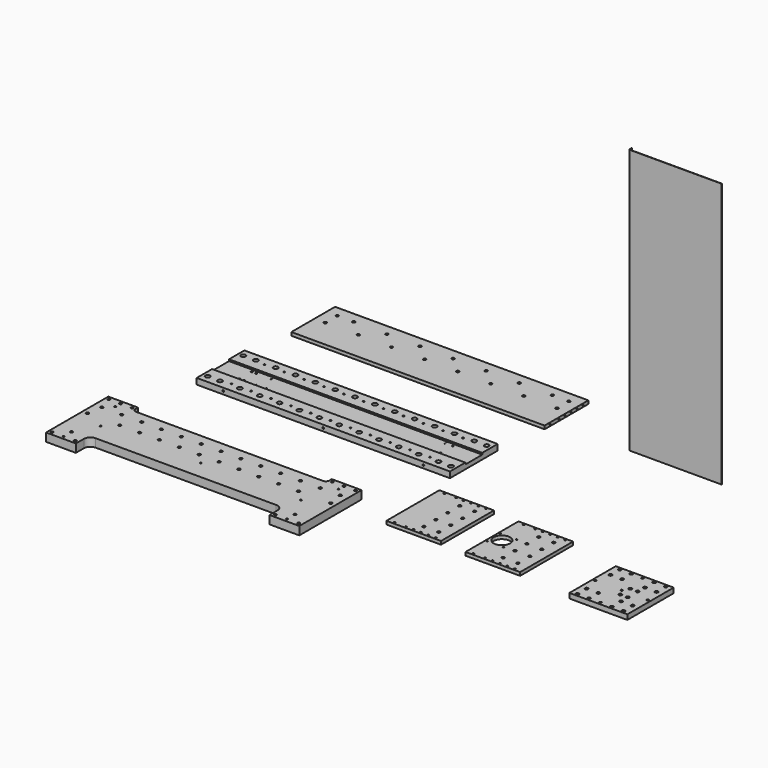
from build123d import *

# Parameters (mm, degrees)
F0_W            = 765
F0_H            = 180
F0_R            = 2.5
F1_DEPTH        = 18
F0_H_2          = 165
F2_DEPTH        = 10
F4_R            = 2.1
F5_DEPTH        = 15
F6_R            = 2.1
F7_DEPTH        = 15
F0_W_2          = 165
F0_H_3          = 200
F0_R_2          = 2.65
F8_DEPTH        = 10
F9_DEPTH        = 10
F0_W_3          = 175
F0_H_4          = 175
F0_R_3          = 4.75
F0_R_4          = 3.35
F0_R_5          = 3
F10_DEPTH       = 15
F11_DEPTH       = 9
F12_W           = 765
F12_H           = 64
F12_R           = 2.5
F13_DEPTH       = 5
F14_DEPTH       = 9.3
F15_DEPTH       = 25
F17_D           = 7.5
F18_D           = 5
F19_DEPTH       = 800
F20_D           = 50
F21_D           = 4.2
F22_D           = 8.4
F23_D           = 8.4
F25_D           = 8.4
F25_CBORE_D     = 14
F25_CBORE_DEPTH = 9
F27_D           = 8.4
F27_CBORE_D     = 14
F27_CBORE_DEPTH = 11
F28_D           = 8.4
F30_D           = 2.5
F32_D           = 5
F32_DEPTH       = 12
F32_TIP         = 1.5021515476
F33_D           = 4.99
F33_DEPTH       = 10
F33_TIP         = 1.4991472445


# Not quite as in the source:
# - a feature names something its author has since deleted; it is built from what else it names


with BuildPart() as f1:
    # F0 (on Top) → F1 (new body)
    with BuildSketch(Plane.XY):
        with Locations((62.1241629124, -27)):
            Rectangle(F0_W, F0_H)
        with Locations((-237.8758370876, -89.5)):
            Circle(F0_R, mode=Mode.SUBTRACT)
        with Locations((-244.3758370876, -50)):
            Circle(F0_R, mode=Mode.SUBTRACT)
        with Locations((-231.3758370876, -50)):
            Circle(F0_R, mode=Mode.SUBTRACT)
        with Locations((-244.3758370876, -4)):
            Circle(F0_R, mode=Mode.SUBTRACT)
        with Locations((-231.3758370876, -4)):
            Circle(F0_R, mode=Mode.SUBTRACT)
        with Locations((-177.8758370876, -89.5)):
            Circle(F0_R, mode=Mode.SUBTRACT)
        with Locations((-117.8758370876, -89.5)):
            Circle(F0_R, mode=Mode.SUBTRACT)
        with Locations((-57.8758370876, -89.5)):
            Circle(F0_R, mode=Mode.SUBTRACT)
        with Locations((-237.8758370876, 35.5)):
            Circle(F0_R, mode=Mode.SUBTRACT)
        with Locations((-177.8758370876, 35.5)):
            Circle(F0_R, mode=Mode.SUBTRACT)
        with Locations((-117.8758370876, 35.5)):
            Circle(F0_R, mode=Mode.SUBTRACT)
        with Locations((-57.8758370876, 35.5)):
            Circle(F0_R, mode=Mode.SUBTRACT)
        with Locations((2.1241629124, -89.5)):
            Circle(F0_R, mode=Mode.SUBTRACT)
        with Locations((62.1241629124, -89.5)):
            Circle(F0_R, mode=Mode.SUBTRACT)
        with Locations((122.1241629124, -89.5)):
            Circle(F0_R, mode=Mode.SUBTRACT)
        with Locations((182.1241629124, -89.5)):
            Circle(F0_R, mode=Mode.SUBTRACT)
        with Locations((242.1241629124, -89.5)):
            Circle(F0_R, mode=Mode.SUBTRACT)
        with Locations((302.1241629124, -89.5)):
            Circle(F0_R, mode=Mode.SUBTRACT)
        with Locations((362.1241629124, -89.5)):
            Circle(F0_R, mode=Mode.SUBTRACT)
        with Locations((362.6241629124, -50)):
            Circle(F0_R, mode=Mode.SUBTRACT)
        with Locations((362.6241629124, -4)):
            Circle(F0_R, mode=Mode.SUBTRACT)
        with Locations((2.1241629124, 35.5)):
            Circle(F0_R, mode=Mode.SUBTRACT)
        with Locations((62.1241629124, 35.5)):
            Circle(F0_R, mode=Mode.SUBTRACT)
        with Locations((122.1241629124, 35.5)):
            Circle(F0_R, mode=Mode.SUBTRACT)
        with Locations((182.1241629124, 35.5)):
            Circle(F0_R, mode=Mode.SUBTRACT)
        with Locations((242.1241629124, 35.5)):
            Circle(F0_R, mode=Mode.SUBTRACT)
        with Locations((302.1241629124, 35.5)):
            Circle(F0_R, mode=Mode.SUBTRACT)
        with Locations((362.1241629124, 35.5)):
            Circle(F0_R, mode=Mode.SUBTRACT)
    extrude(amount=F1_DEPTH)

    # F12 (on face) → F13 (cut)
    with BuildSketch(Plane.XY.offset(18)):
        with Locations((62.1241629124, -27)):
            Rectangle(F12_W, F12_H)
        with Locations((-244.3758370876, -50)):
            Circle(F12_R, mode=Mode.SUBTRACT)
        with Locations((-231.3758370876, -50)):
            Circle(F12_R, mode=Mode.SUBTRACT)
        with Locations((362.6241629124, -50)):
            Circle(F12_R, mode=Mode.SUBTRACT)
        with Locations((-244.3758370876, -4)):
            Circle(F12_R, mode=Mode.SUBTRACT)
        with Locations((-231.3758370876, -4)):
            Circle(F12_R, mode=Mode.SUBTRACT)
        with Locations((362.6241629124, -4)):
            Circle(F12_R, mode=Mode.SUBTRACT)
    extrude(amount=-F13_DEPTH, mode=Mode.SUBTRACT)

    # F25 (through all)
    with Locations(Plane.XY.offset(18)):
        with Locations((-305.3758370876, 40.5), (-305.3758370876, -94.5), (-267.8758370876, 40.5), (-267.8758370876, -94.5), (-207.8758370876, 40.5), (-207.8758370876, -94.5), (-147.8758370876, 40.5), (-147.8758370876, -94.5), (-87.8758370876, 40.5), (-87.8758370876, -94.5), (-27.8758370876, 40.5), (-27.8758370876, -94.5), (32.1241629124, -94.5), (92.1241629124, -94.5), (152.1241629124, -94.5), (212.1241629124, -94.5), (32.1241629124, 40.5), (92.1241629124, 40.5), (152.1241629124, 40.5), (212.1241629124, 40.5), (272.1241629124, 40.5), (332.1241629124, 40.5), (392.1241629124, 40.5), (429.6241629124, 40.5), (272.1241629124, -94.5), (332.1241629124, -94.5), (392.1241629124, -94.5), (429.6241629124, -94.5)):
            CounterBoreHole(F25_D / 2, F25_CBORE_D / 2, F25_CBORE_DEPTH)

    # F30 (through all)
    with Locations(Plane.XY.offset(13)):
        with Locations((-185.3758370876, 1), (-185.3758370876, -6), (-195.3758370876, -48), (-195.3758370876, -55), (-165.3758370876, -47.9999991988), (-165.3758370876, -55), (339.6241629124, 1), (339.6241629124, -6)):
            Hole(F30_D / 2)

    # F32
    with Locations(Plane.XZ.offset(117)):
        with Locations((-240.3758370876, 9), (62.1241629124, 9), (364.6241629124, 9)):
            Hole(F32_D / 2, depth=F32_DEPTH)
            with Locations((0, 0, -(F32_DEPTH + F32_TIP / 2))):  # 118° drill point
                Cone(0, F32_D / 2, F32_TIP, mode=Mode.SUBTRACT)


with BuildPart() as f2:
    # F0 (on Top) → F2 (new body)
    with BuildSketch(Plane.XY):
        with Locations((80.4346650839, 300.0778406858)):
            Rectangle(F0_W, F0_H_2)
    extrude(amount=F2_DEPTH)

    # F4 (on face) → F5 (cut)
    with BuildSketch(Plane.YZ.offset(462.9346650839)):
        with Locations((237.5778406858, 5)):
            Circle(F4_R)
        with Locations((272.5778406858, 5)):
            Circle(F4_R)
        with Locations((295.0778406858, 5)):
            Circle(F4_R)
        with Locations((317.5778406858, 5)):
            Circle(F4_R)
        with Locations((340.0778406858, 5)):
            Circle(F4_R)
        with Locations((362.5778406858, 5)):
            Circle(F4_R)
    extrude(amount=-F5_DEPTH, mode=Mode.SUBTRACT)

    # F6 (on face) → F7 (cut)
    with BuildSketch(Plane(origin=(-302.0653349161, 0, 0), x_dir=(0, -1, 0), z_dir=(-1, 0, 0))):
        with Locations((-237.5778406858, 5)):
            Circle(F6_R)
        with Locations((-272.5778406858, 5)):
            Circle(F6_R)
        with Locations((-295.0778406858, 5)):
            Circle(F6_R)
        with Locations((-317.5778406858, 5)):
            Circle(F6_R)
        with Locations((-340.0778406858, 5)):
            Circle(F6_R)
        with Locations((-362.5778406858, 5)):
            Circle(F6_R)
    extrude(amount=-F7_DEPTH, mode=Mode.SUBTRACT)

    # F28 (through all)
    with Locations(Plane.XY.offset(10)):
        with Locations((-269.5653349161, 350.0778406858), (-269.5653349161, 305.0778406858), (-219.5653349161, 350.0778406858), (-169.5653349161, 305.0778406858), (-119.5653349161, 350.0778406858), (-69.5653349161, 305.0778406858), (-19.5653349161, 350.0778406858), (30.4346650839, 305.0778406858), (80.4346650839, 350.0778406858), (130.4346650839, 305.0778406858), (180.4346650839, 350.0778406858), (230.4346650839, 305.0778406858), (280.4346650839, 350.0778406858), (330.4346650839, 305.0778406858), (380.4346650839, 350.0778406858), (430.4346650839, 350.0778406858), (430.4346650839, 305.0778406858)):
            Hole(F28_D / 2)


with BuildPart() as f8:
    # F0 (on Top) → F8 (new body)
    with BuildSketch(Plane.XY):
        with Locations((557.9147299131, -295.5082142353)):
            Rectangle(F0_W_2, F0_H_3)
        with Locations((495.4147299131, -390.5082142353)):
            Circle(F0_R_2, mode=Mode.SUBTRACT)
        with Locations((530.4147299131, -390.5082142353)):
            Circle(F0_R_2, mode=Mode.SUBTRACT)
        with Locations((552.9147299131, -390.5082142353)):
            Circle(F0_R_2, mode=Mode.SUBTRACT)
        with Locations((575.4147299131, -390.5082142353)):
            Circle(F0_R_2, mode=Mode.SUBTRACT)
        with Locations((597.9147299131, -390.5082142353)):
            Circle(F0_R_2, mode=Mode.SUBTRACT)
        with Locations((620.4147299131, -390.5082142353)):
            Circle(F0_R_2, mode=Mode.SUBTRACT)
        with Locations((495.4147299131, -200.5082142353)):
            Circle(F0_R_2, mode=Mode.SUBTRACT)
        with Locations((530.4147299131, -200.5082142353)):
            Circle(F0_R_2, mode=Mode.SUBTRACT)
        with Locations((552.9147299131, -200.5082142353)):
            Circle(F0_R_2, mode=Mode.SUBTRACT)
        with Locations((575.4147299131, -200.5082142353)):
            Circle(F0_R_2, mode=Mode.SUBTRACT)
        with Locations((597.9147299131, -200.5082142353)):
            Circle(F0_R_2, mode=Mode.SUBTRACT)
        with Locations((620.4147299131, -200.5082142353)):
            Circle(F0_R_2, mode=Mode.SUBTRACT)
    extrude(amount=F8_DEPTH)

    # F23 (through all)
    with Locations(Plane(origin=(0, 0, 0), x_dir=(1, 0, 0), z_dir=(0, 0, -1))):
        with Locations((607.9147299131, 228.0082142353), (562.9147299131, 228.0082142353), (607.9147299131, 273.0082142353), (562.9147299131, 273.0082142353), (607.9147299131, 318.0082142353), (562.9147299131, 318.0082142353), (607.9147299131, 363.0082142353), (562.9147299131, 363.0082142353)):
            Hole(F23_D / 2)


with BuildPart() as f9:
    # F0 (on Top) → F9 (new body)
    with BuildSketch(Plane.XY):
        Polygon((720.5080483251, -303.1488111544), (720.5080483251, -403.1488111544), (885.5080483251, -403.1488111544), (885.5080483251, -203.1488111544), (720.5080483251, -203.1488111544), align=None)
        with Locations((740.5080483251, -398.1488111544)):
            Circle(F0_R_2, mode=Mode.SUBTRACT)
        with Locations((775.5080483251, -398.1488111544)):
            Circle(F0_R_2, mode=Mode.SUBTRACT)
        with Locations((798.0080483251, -398.1488111544)):
            Circle(F0_R_2, mode=Mode.SUBTRACT)
        with Locations((820.5080483251, -398.1488111544)):
            Circle(F0_R_2, mode=Mode.SUBTRACT)
        with Locations((843.0080483251, -398.1488111544)):
            Circle(F0_R_2, mode=Mode.SUBTRACT)
        with Locations((865.5080483251, -398.1488111544)):
            Circle(F0_R_2, mode=Mode.SUBTRACT)
        with Locations((740.5080483251, -208.1488111544)):
            Circle(F0_R_2, mode=Mode.SUBTRACT)
        with Locations((775.5080483251, -208.1488111544)):
            Circle(F0_R_2, mode=Mode.SUBTRACT)
        with Locations((798.0080483251, -208.1488111544)):
            Circle(F0_R_2, mode=Mode.SUBTRACT)
        with Locations((820.5080483251, -208.1488111544)):
            Circle(F0_R_2, mode=Mode.SUBTRACT)
        with Locations((843.0080483251, -208.1488111544)):
            Circle(F0_R_2, mode=Mode.SUBTRACT)
        with Locations((865.5080483251, -208.1488111544)):
            Circle(F0_R_2, mode=Mode.SUBTRACT)
    extrude(amount=F9_DEPTH)

    # F20 (through all)
    with Locations(Plane(origin=(0, 0, 0), x_dir=(1, 0, 0), z_dir=(0, 0, -1))):
        with Locations((750.5080483251, 303.1488111544)):
            Hole(F20_D / 2)

    # F21 (through all)
    with Locations(Plane(origin=(0, 0, 0), x_dir=(1, 0, 0), z_dir=(0, 0, -1))):
        with Locations((775.2567856666, 278.4000738129), (725.7593109836, 278.4000738129), (775.2567856666, 327.8975484959), (725.7593109836, 327.8975484959)):
            Hole(F21_D / 2)

    # F22 (through all)
    with Locations(Plane(origin=(0, 0, 0), x_dir=(1, 0, 0), z_dir=(0, 0, -1))):
        with Locations((853.0080483251, 235.6488111544), (808.0080483251, 235.6488111544), (808.0080483251, 280.6488111544), (853.0080483251, 280.6488111544), (853.0080483251, 325.6488111544), (808.0080483251, 325.6488111544), (808.0080483251, 370.6488111544), (853.0080483251, 370.6488111544)):
            Hole(F22_D / 2)


with BuildPart() as f10:
    # F0 (on Top) → F10 (new body)
    with BuildSketch(Plane.XY):
        with Locations((1136.3020181656, -333.5187590122)):
            Rectangle(F0_W_3, F0_H_4)
        with Locations((1066.8020181656, -413.5187590122)):
            Circle(F0_R_3, mode=Mode.SUBTRACT)
        with Locations((1101.8020181656, -413.5187590122)):
            Circle(F0_R_3, mode=Mode.SUBTRACT)
        with Locations((1136.3020181656, -413.0187590122)):
            Circle(F0_R_4, mode=Mode.SUBTRACT)
        with Locations((1170.8020181656, -413.5187590122)):
            Circle(F0_R_3, mode=Mode.SUBTRACT)
        with Locations((1205.8020181656, -413.5187590122)):
            Circle(F0_R_3, mode=Mode.SUBTRACT)
        with Locations((1066.8020181656, -378.5187590122)):
            Circle(F0_R_3, mode=Mode.SUBTRACT)
        with Locations((1101.8020181656, -378.5187590122)):
            Circle(F0_R_3, mode=Mode.SUBTRACT)
        with Locations((1056.8020181656, -333.5187590122)):
            Circle(F0_R_4, mode=Mode.SUBTRACT)
        with Locations((1170.8020181656, -378.5187590122)):
            Circle(F0_R_3, mode=Mode.SUBTRACT)
        with Locations((1205.8020181656, -378.5187590122)):
            Circle(F0_R_3, mode=Mode.SUBTRACT)
        with Locations((1147.8020181656, -352.5187590122)):
            Circle(F0_R_3, mode=Mode.SUBTRACT)
        with Locations((1169.8020181656, -352.5187590122)):
            Circle(F0_R_3, mode=Mode.SUBTRACT)
        with Locations((1136.3020181656, -333.5187590122)):
            Circle(F0_R_5, mode=Mode.SUBTRACT)
        with Locations((1215.8020181656, -333.5187590122)):
            Circle(F0_R_4, mode=Mode.SUBTRACT)
        with Locations((1066.8020181656, -288.5187590122)):
            Circle(F0_R_3, mode=Mode.SUBTRACT)
        with Locations((1101.8020181656, -288.5187590122)):
            Circle(F0_R_3, mode=Mode.SUBTRACT)
        with Locations((1147.8020181656, -314.5187590122)):
            Circle(F0_R_3, mode=Mode.SUBTRACT)
        with Locations((1169.8020181656, -314.5187590122)):
            Circle(F0_R_3, mode=Mode.SUBTRACT)
        with Locations((1170.8020181656, -288.5187590122)):
            Circle(F0_R_3, mode=Mode.SUBTRACT)
        with Locations((1205.8020181656, -288.5187590122)):
            Circle(F0_R_3, mode=Mode.SUBTRACT)
        with Locations((1066.8020181656, -253.5187590122)):
            Circle(F0_R_3, mode=Mode.SUBTRACT)
        with Locations((1101.8020181656, -253.5187590122)):
            Circle(F0_R_3, mode=Mode.SUBTRACT)
        with Locations((1136.3020181656, -254.0187590122)):
            Circle(F0_R_4, mode=Mode.SUBTRACT)
        with Locations((1170.8020181656, -253.5187590122)):
            Circle(F0_R_3, mode=Mode.SUBTRACT)
        with Locations((1205.8020181656, -253.5187590122)):
            Circle(F0_R_3, mode=Mode.SUBTRACT)
    extrude(amount=F10_DEPTH)

    # F0 (on Top) → F11 (join)
    with BuildSketch(Plane.XY):
        with Locations((1147.8020181656, -314.5187590122)):
            Circle(F0_R_3)
        with Locations((1147.8020181656, -314.5187590122)):
            Circle(F0_R_2, mode=Mode.SUBTRACT)
        with Locations((1169.8020181656, -314.5187590122)):
            Circle(F0_R_3)
        with Locations((1169.8020181656, -314.5187590122)):
            Circle(F0_R_2, mode=Mode.SUBTRACT)
        with Locations((1147.8020181656, -352.5187590122)):
            Circle(F0_R_3)
        with Locations((1147.8020181656, -352.5187590122)):
            Circle(F0_R_2, mode=Mode.SUBTRACT)
        with Locations((1169.8020181656, -352.5187590122)):
            Circle(F0_R_3)
        with Locations((1169.8020181656, -352.5187590122)):
            Circle(F0_R_2, mode=Mode.SUBTRACT)
    extrude(amount=F11_DEPTH)

    # F0 (on Top) → F14 (join)
    with BuildSketch(Plane.XY):
        with Locations((1066.8020181656, -253.5187590122)):
            Circle(F0_R_3)
        with Locations((1066.8020181656, -253.5187590122)):
            Circle(F0_R_2, mode=Mode.SUBTRACT)
        with Locations((1101.8020181656, -253.5187590122)):
            Circle(F0_R_3)
        with Locations((1101.8020181656, -253.5187590122)):
            Circle(F0_R_2, mode=Mode.SUBTRACT)
        with Locations((1066.8020181656, -288.5187590122)):
            Circle(F0_R_3)
        with Locations((1066.8020181656, -288.5187590122)):
            Circle(F0_R_2, mode=Mode.SUBTRACT)
        with Locations((1101.8020181656, -288.5187590122)):
            Circle(F0_R_3)
        with Locations((1101.8020181656, -288.5187590122)):
            Circle(F0_R_2, mode=Mode.SUBTRACT)
        with Locations((1170.8020181656, -253.5187590122)):
            Circle(F0_R_3)
        with Locations((1170.8020181656, -253.5187590122)):
            Circle(F0_R_2, mode=Mode.SUBTRACT)
        with Locations((1205.8020181656, -253.5187590122)):
            Circle(F0_R_3)
        with Locations((1205.8020181656, -253.5187590122)):
            Circle(F0_R_2, mode=Mode.SUBTRACT)
        with Locations((1205.8020181656, -288.5187590122)):
            Circle(F0_R_3)
        with Locations((1205.8020181656, -288.5187590122)):
            Circle(F0_R_2, mode=Mode.SUBTRACT)
        with Locations((1170.8020181656, -288.5187590122)):
            Circle(F0_R_3)
        with Locations((1170.8020181656, -288.5187590122)):
            Circle(F0_R_2, mode=Mode.SUBTRACT)
        with Locations((1205.8020181656, -378.5187590122)):
            Circle(F0_R_3)
        with Locations((1205.8020181656, -378.5187590122)):
            Circle(F0_R_2, mode=Mode.SUBTRACT)
        with Locations((1170.8020181656, -378.5187590122)):
            Circle(F0_R_3)
        with Locations((1170.8020181656, -378.5187590122)):
            Circle(F0_R_2, mode=Mode.SUBTRACT)
        with Locations((1170.8020181656, -413.5187590122)):
            Circle(F0_R_3)
        with Locations((1170.8020181656, -413.5187590122)):
            Circle(F0_R_2, mode=Mode.SUBTRACT)
        with Locations((1205.8020181656, -413.5187590122)):
            Circle(F0_R_3)
        with Locations((1205.8020181656, -413.5187590122)):
            Circle(F0_R_2, mode=Mode.SUBTRACT)
        with Locations((1066.8020181656, -378.5187590122)):
            Circle(F0_R_3)
        with Locations((1066.8020181656, -378.5187590122)):
            Circle(F0_R_2, mode=Mode.SUBTRACT)
        with Locations((1101.8020181656, -378.5187590122)):
            Circle(F0_R_3)
        with Locations((1101.8020181656, -378.5187590122)):
            Circle(F0_R_2, mode=Mode.SUBTRACT)
        with Locations((1101.8020181656, -413.5187590122)):
            Circle(F0_R_3)
        with Locations((1101.8020181656, -413.5187590122)):
            Circle(F0_R_2, mode=Mode.SUBTRACT)
        with Locations((1066.8020181656, -413.5187590122)):
            Circle(F0_R_3)
        with Locations((1066.8020181656, -413.5187590122)):
            Circle(F0_R_2, mode=Mode.SUBTRACT)
    extrude(amount=F14_DEPTH)


with BuildPart() as f15:
    # F0 (on Top) → F15 (new body)
    with BuildSketch(Plane.XY):
        with BuildLine():
            Line((-325.3115415573, -332.1774768829), (-415.3115415573, -332.1774768829))
            Line((-415.3115415573, -332.1774768829), (-415.3115415573, -567.1774768829))
            Line((-415.3115415573, -567.1774768829), (-325.3115415573, -567.1774768829))
            Line((-325.3115415573, -567.1774768829), (-325.3115415573, -537.1774768829))
            ThreePointArc((-325.3115415573, -537.1774768829), (-319.453677181, -523.0353412592), (-305.3115415573, -517.1774768829))
            Line((-305.3115415573, -517.1774768829), (239.6884584427, -517.1774768829))
            ThreePointArc((239.6884584427, -517.1774768829), (253.8305940664, -523.0353412592), (259.6884584427, -537.1774768829))
            Line((259.6884584427, -537.1774768829), (259.6884584427, -567.1774768829))
            Line((259.6884584427, -567.1774768829), (349.6884584427, -567.1774768829))
            Line((349.6884584427, -567.1774768829), (349.6884584427, -332.1774768829))
            Line((349.6884584427, -332.1774768829), (259.6884584427, -332.1774768829))
            Line((259.6884584427, -332.1774768829), (259.6884584427, -342.1774768829))
            ThreePointArc((259.6884584427, -342.1774768829), (256.7595262546, -349.2485446948), (249.6884584427, -352.1774768829))
            Line((249.6884584427, -352.1774768829), (-315.3115415573, -352.1774768829))
            ThreePointArc((-315.3115415573, -352.1774768829), (-322.3826093692, -349.2485446948), (-325.3115415573, -342.1774768829))
            Line((-325.3115415573, -342.1774768829), (-325.3115415573, -332.1774768829))
        make_face()
    extrude(amount=F15_DEPTH)

    # F17 (through all)
    with Locations(Plane.XY.offset(25)):
        with Locations((-405.3115415573, -342.1774768829), (-370.3115415573, -342.1774768829), (-405.3115415573, -557.1774768829), (-370.3115415573, -527.1774768829), (-335.3115415573, -557.1774768829), (269.6884584427, -557.1774768829), (304.6884584427, -527.1774768829), (339.6884584427, -557.1774768829), (304.6884584427, -342.1774768829), (339.6884584427, -342.1774768829), (-335.3115415573, -342.1774768829), (269.6884584427, -342.1774768829)):
            Hole(F17_D / 2)

    # F18 (through all)
    with Locations(Plane.XY.offset(25)):
        with Locations((-370.3115415573, -362.1774768829), (304.6884584427, -362.1774768829), (-370.3115415573, -557.1774768829), (304.6884584427, -557.1774768829)):
            Hole(F18_D / 2)

    # F27 (through all)
    with Locations(Plane(origin=(0, 0, 0), x_dir=(1, 0, 0), z_dir=(0, 0, -1))):
        with Locations((334.6884584427, 429.6774768829), (327.1884584427, 384.6774768829), (267.1884584427, 384.6774768829), (237.1884584427, 429.6774768829), (207.1884584427, 384.6774768829), (177.1884584427, 429.6774768829), (147.1884584427, 384.6774768829), (117.1884584427, 429.6774768829), (87.1884584427, 384.6774768829), (57.1884584427, 429.6774768829), (27.1884584427, 384.6774768829), (-2.8115415573, 429.6774768829), (-32.8115415573, 384.6774768829), (-62.8115415573, 429.6774768829), (-92.8115415573, 384.6774768829), (-122.8115415573, 429.6774768829), (-182.8115415573, 429.6774768829), (-242.8115415573, 429.6774768829), (-302.8115415573, 429.6774768829), (-272.8115415573, 384.6774768829), (-212.8115415573, 384.6774768829), (-152.8115415573, 384.6774768829), (-332.8115415573, 384.6774768829), (-392.8115415573, 384.6774768829), (-400.3115415573, 429.6774768829)):
            CounterBoreHole(F27_D / 2, F27_CBORE_D / 2, F27_CBORE_DEPTH)

    # F33
    with Locations(Plane.XY.offset(25)):
        with Locations((-335.3115415573, -461.1774768829), (-32.8115415573, -461.1774768829), (269.6884584427, -461.1774768829)):
            Hole(F33_D / 2, depth=F33_DEPTH)
            with Locations((0, 0, -(F33_DEPTH + F33_TIP / 2))):  # 118° drill point
                Cone(0, F33_D / 2, F33_TIP, mode=Mode.SUBTRACT)


with BuildPart() as f19:
    # F0 (on Top) → F19 (new body)
    with BuildSketch(Plane.XY):
        with BuildLine():
            Line((686.4871172905, 267.9644193649), (685.4871172905, 267.9644193649))
            Line((685.4871172905, 267.9644193649), (685.4871172905, 260.9644193649))
            ThreePointArc((685.4871172905, 260.9644193649), (686.3657969469, 258.8430990214), (688.4871172905, 257.9644193649))
            Line((688.4871172905, 257.9644193649), (965.4871172905, 257.9644193649))
            Line((965.4871172905, 257.9644193649), (965.4871172905, 258.9644193649))
            Line((965.4871172905, 258.9644193649), (689.4871172905, 258.9644193649))
            ThreePointArc((689.4871172905, 258.9644193649), (687.3657969469, 259.8430990214), (686.4871172905, 261.9644193649))
            Line((686.4871172905, 261.9644193649), (686.4871172905, 267.9644193649))
        make_face()
    extrude(amount=F19_DEPTH)


solid = Compound([f1.part, f2.part, f8.part, f9.part, f10.part, f15.part, f19.part])
